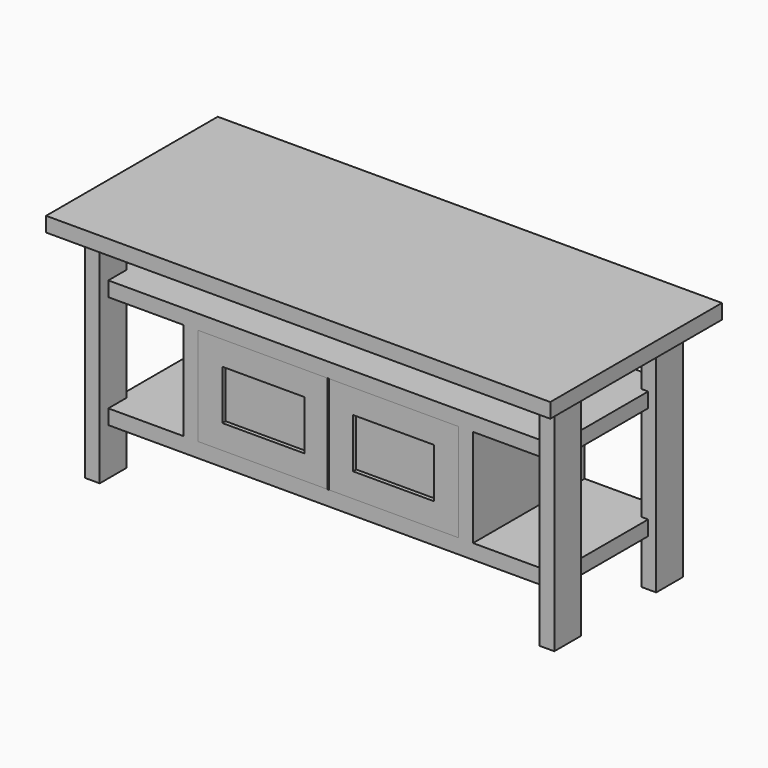
from build123d import *

# Parameters (mm, degrees)
F1_DEPTH      = 254
F0_W          = 615.95
F0_H          = 231.775
F2_DEPTH      = 165.1
F2_DEPTH_BACK = 165.1
F0_W_2        = 15.875
F0_H_2        = 38.1
F3_W          = 34.925
F3_H          = 79.375
F4_DEPTH      = 523.875
F5_W          = 306.3875
F5_H          = 231.775
F5_W_2        = 195.2625
F5_H_2        = 117.475
F6_DEPTH      = 34.925
F5_W_3        = 192.0875
F7_DEPTH      = 9.525


with BuildPart() as f1:
    # F0 (on Front) → F1 (new body, symmetric)
    with BuildSketch(Plane.XZ):
        Polygon((596.9, 523.875), (596.9, 558.8), (-596.9, 558.8), (-596.9, 523.875), (-536.575, 523.875), (-520.7, 523.875), (-495.3, 523.875), (-479.425, 523.875), (479.425, 523.875), (495.3, 523.875), (520.7, 523.875), (536.575, 523.875), align=None)
    extrude(amount=F1_DEPTH, both=True)

    # F0 (on Front) → F2, piece 3 (join, two sides)
    with BuildSketch(Plane.XZ) as f2_3_sk:
        with Locations((487.3625, 504.825)):
            Rectangle(F0_W_2, F0_H_2)
        with Locations((-487.3625, 504.825)):
            Rectangle(F0_W_2, F0_H_2)
    extrude(amount=F2_DEPTH)
    extrude(f2_3_sk.sketch, amount=-F2_DEPTH_BACK)


with BuildPart() as f2:
    # F0 (on Front) → F2 (new body, two sides)
    with BuildSketch(Plane.XZ) as f2_sk:
        Polygon((536.575, 111.125), (536.575, 146.05), (342.9, 146.05), (342.9, 377.825), (536.575, 377.825), (536.575, 412.75), (-536.575, 412.75), (-536.575, 377.825), (-342.9, 377.825), (-342.9, 146.05), (-536.575, 146.05), (-536.575, 111.125), align=None)
        with Locations((0, 261.9375)):
            Rectangle(F0_W, F0_H, mode=Mode.SUBTRACT)
    extrude(amount=F2_DEPTH)
    extrude(f2_sk.sketch, amount=-F2_DEPTH_BACK)



with BuildPart() as f2b:
    # F0 (on Front) → F2, piece 2 (new body, two sides)
    with BuildSketch(Plane.XZ) as f2_2_sk:
        with Locations((528.6375, 504.825)):
            Rectangle(F0_W_2, F0_H_2)
    extrude(amount=F2_DEPTH)
    extrude(f2_2_sk.sketch, amount=-F2_DEPTH_BACK)


with BuildPart() as f2c:
    # F0 (on Front) → F2, piece 4 (new body, two sides)
    with BuildSketch(Plane.XZ) as f2_4_sk:
        with Locations((-528.6375, 504.825)):
            Rectangle(F0_W_2, F0_H_2)
    extrude(amount=F2_DEPTH)
    extrude(f2_4_sk.sketch, amount=-F2_DEPTH_BACK)


with BuildPart() as f2_1:
    add(f2.part)

    add(f2b.part)  # F4 merges F2b

    add(f2c.part)  # F4 merges F2c
    # F3 (on Top) → F4 (join, through all)
    with BuildSketch(Plane.XY):
        with Locations((-538.1625, 150.8125)):
            Rectangle(F3_W, F3_H)
        with Locations((-538.1625, -150.8125)):
            Rectangle(F3_W, F3_H)
        with Locations((538.1625, -150.8125)):
            Rectangle(F3_W, F3_H)
        with Locations((538.1625, 150.8125)):
            Rectangle(F3_W, F3_H)
    extrude(amount=F4_DEPTH)


with BuildPart() as f6:
    # F5 (on face) → F6 (new body)
    with BuildSketch(Plane.XZ.offset(165.1)):
        with Locations((-154.78125, 261.9375)):
            Rectangle(F5_W, F5_H)
        with Locations((-153.19375, 261.9375)):
            Rectangle(F5_W_2, F5_H_2, mode=Mode.SUBTRACT)
        with Locations((-153.19375, 261.9375)):
            Rectangle(F5_W_2, F5_H_2)
    extrude(amount=-F6_DEPTH)


with BuildPart() as f6b:
    # F5 (on face) → F6, piece 2 (new body)
    with BuildSketch(Plane.XZ.offset(165.1)):
        with Locations((154.78125, 261.9375)):
            Rectangle(F5_W, F5_H)
        with Locations((154.78125, 261.9375)):
            Rectangle(F5_W_3, F5_H_2, mode=Mode.SUBTRACT)
        with Locations((154.78125, 261.9375)):
            Rectangle(F5_W_3, F5_H_2)
    extrude(amount=-F6_DEPTH)


with BuildPart() as f7_tool:
    # F5 (on face) → F7 (new body)
    with BuildSketch(Plane.XZ.offset(165.1)):
        with Locations((-153.19375, 261.9375)):
            Rectangle(F5_W_2, F5_H_2)
        with Locations((154.78125, 261.9375)):
            Rectangle(F5_W_3, F5_H_2)
    extrude(amount=-F7_DEPTH)


with BuildPart() as f6_1:
    add(f6.part)

    # F7: cut by f7_tool
    add(f7_tool.part, mode=Mode.SUBTRACT)


with BuildPart() as f6b_1:
    add(f6b.part)

    # F7: cut by f7_tool
    add(f7_tool.part, mode=Mode.SUBTRACT)


with BuildPart() as f8_1:
    # F8: instance of F6
    add(f6_1.part.mirror(Plane.XZ))


with BuildPart() as f8_2:
    # F8: instance of F6b
    add(f6b_1.part.mirror(Plane.XZ))


solid = Compound([f1.part, f2_1.part, f6_1.part, f6b_1.part, f8_1.part, f8_2.part])
